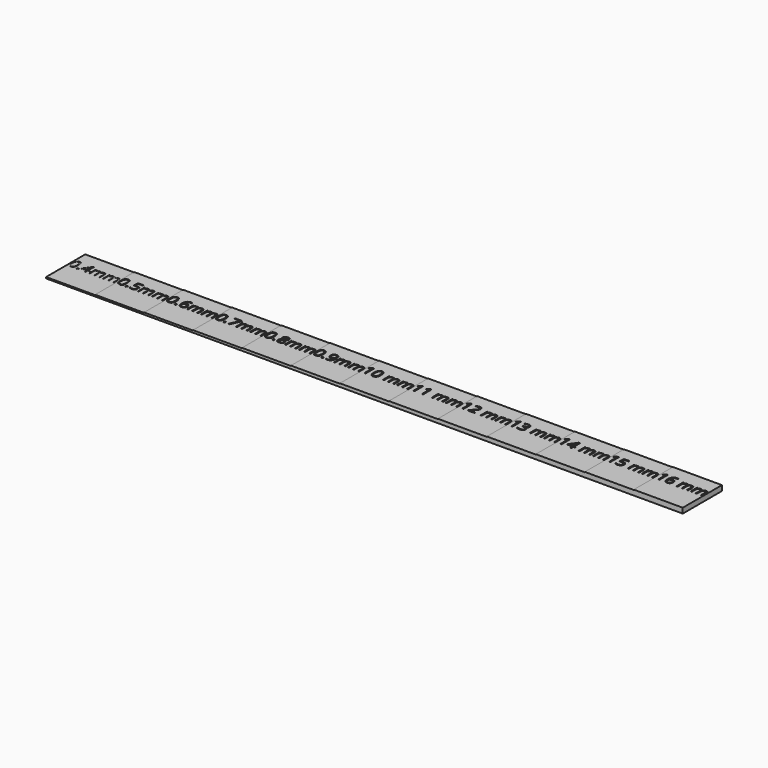
from build123d import *

# Parameters (mm, degrees)
F0_W          = 15
F0_H          = 15
F1_DEPTH      = 0.4
F2_DEPTH      = 0.5
F3_DEPTH      = 0.6
F4_DEPTH      = 0.7
F5_DEPTH      = 0.8
F6_DEPTH      = 0.9
F7_DEPTH      = 1
F8_DEPTH      = 1.1
F9_DEPTH      = 1.2
F10_DEPTH     = 1.3
F11_DEPTH     = 1.4
F12_DEPTH     = 1.5
F13_DEPTH     = 1.6
F14_TEXT_SIZE = 4.6102867022
F15_DEPTH     = 0.1
F16_TEXT_SIZE = 4.6102867022
F17_DEPTH     = 0.2
F18_TEXT_SIZE = 4.6102867022
F19_DEPTH     = 0.3
F20_TEXT_SIZE = 4.6102867022
F21_DEPTH     = 0.4
F22_TEXT_SIZE = 4.6102867022
F23_DEPTH     = 0.5
F24_TEXT_SIZE = 4.6102867022
F25_DEPTH     = 0.6
F26_TEXT_SIZE = 4.6191598903
F27_DEPTH     = 0.7
F28_TEXT_SIZE = 4.6191598903
F29_DEPTH     = 0.8
F30_TEXT_SIZE = 4.6191598903
F31_DEPTH     = 0.9
F32_TEXT_SIZE = 4.6191598903
F33_DEPTH     = 1
F34_TEXT_SIZE = 4.6191598903
F35_DEPTH     = 1.1
F36_TEXT_SIZE = 4.6191598903
F37_DEPTH     = 1.2
F38_TEXT_SIZE = 4.6191598903
F39_DEPTH     = 1.3


# Not quite as in the source:
# - Text() gives the source's letters only with a copy of the font that has no kerning and outlines rounded to 1/6400 em; it was checked with that copy


with BuildPart() as f1:
    # F0 (on Top) → F1 (new body)
    with BuildSketch(Plane.XY):
        with Locations((-77.3718157444, -0.2832734026)):
            Rectangle(F0_W, F0_H)
    extrude(amount=F1_DEPTH)

    # F0 (on Top) → F2 (join)
    with BuildSketch(Plane.XY):
        with Locations((-62.3718157444, -0.2832734026)):
            Rectangle(F0_W, F0_H)
    extrude(amount=F2_DEPTH)

    # F0 (on Top) → F3 (join)
    with BuildSketch(Plane.XY):
        with Locations((-47.3718157444, -0.2832734026)):
            Rectangle(F0_W, F0_H)
    extrude(amount=F3_DEPTH)

    # F0 (on Top) → F4 (join)
    with BuildSketch(Plane.XY):
        with Locations((-32.3718157444, -0.2832734026)):
            Rectangle(F0_W, F0_H)
    extrude(amount=F4_DEPTH)

    # F0 (on Top) → F5 (join)
    with BuildSketch(Plane.XY):
        with Locations((-17.3718157444, -0.2832734026)):
            Rectangle(F0_W, F0_H)
    extrude(amount=F5_DEPTH)

    # F0 (on Top) → F6 (join)
    with BuildSketch(Plane.XY):
        with Locations((-2.3718157444, -0.2832734026)):
            Rectangle(F0_W, F0_H)
    extrude(amount=F6_DEPTH)

    # F0 (on Top) → F7 (join)
    with BuildSketch(Plane.XY):
        with Locations((12.6281842556, -0.2832734026)):
            Rectangle(F0_W, F0_H)
    extrude(amount=F7_DEPTH)

    # F0 (on Top) → F8 (join)
    with BuildSketch(Plane.XY):
        with Locations((27.6281842556, -0.2832734026)):
            Rectangle(F0_W, F0_H)
    extrude(amount=F8_DEPTH)

    # F0 (on Top) → F9 (join)
    with BuildSketch(Plane.XY):
        with Locations((42.6281842556, -0.2832734026)):
            Rectangle(F0_W, F0_H)
    extrude(amount=F9_DEPTH)

    # F0 (on Top) → F10 (join)
    with BuildSketch(Plane.XY):
        with Locations((57.6281842556, -0.2832734026)):
            Rectangle(F0_W, F0_H)
    extrude(amount=F10_DEPTH)

    # F0 (on Top) → F11 (join)
    with BuildSketch(Plane.XY):
        with Locations((72.6281842556, -0.2832734026)):
            Rectangle(F0_W, F0_H)
    extrude(amount=F11_DEPTH)

    # F0 (on Top) → F12 (join)
    with BuildSketch(Plane.XY):
        with Locations((87.6281842556, -0.2832734026)):
            Rectangle(F0_W, F0_H)
    extrude(amount=F12_DEPTH)

    # F0 (on Top) → F13 (join)
    with BuildSketch(Plane.XY):
        with Locations((102.6281842556, -0.2832734026)):
            Rectangle(F0_W, F0_H)
    extrude(amount=F13_DEPTH)

    # F14 (on face) → F15 (cut)
    with BuildSketch(Plane.XY.offset(0.4)):
        with Locations((-84.8718157444, 0)):
            Text('0.4mm', F14_TEXT_SIZE, font='Open Sans', text_align=(TextAlign.LEFT, TextAlign.BOTTOM))
    extrude(amount=-F15_DEPTH, mode=Mode.SUBTRACT)

    # F16 (on face) → F17 (cut)
    with BuildSketch(Plane.XY.offset(0.5)):
        with Locations((-69.8718157444, 0)):
            Text('0.5mm', F16_TEXT_SIZE, font='Open Sans', text_align=(TextAlign.LEFT, TextAlign.BOTTOM))
    extrude(amount=-F17_DEPTH, mode=Mode.SUBTRACT)

    # F18 (on face) → F19 (cut)
    with BuildSketch(Plane.XY.offset(0.6)):
        with Locations((-54.8718157444, 0)):
            Text('0.6mm', F18_TEXT_SIZE, font='Open Sans', text_align=(TextAlign.LEFT, TextAlign.BOTTOM))
    extrude(amount=-F19_DEPTH, mode=Mode.SUBTRACT)

    # F20 (on face) → F21 (cut)
    with BuildSketch(Plane.XY.offset(0.7)):
        with Locations((-39.8718157444, 0)):
            Text('0.7mm', F20_TEXT_SIZE, font='Open Sans', text_align=(TextAlign.LEFT, TextAlign.BOTTOM))
    extrude(amount=-F21_DEPTH, mode=Mode.SUBTRACT)

    # F22 (on face) → F23 (cut)
    with BuildSketch(Plane.XY.offset(0.8)):
        with Locations((-24.8718157444, 0)):
            Text('0.8mm', F22_TEXT_SIZE, font='Open Sans', text_align=(TextAlign.LEFT, TextAlign.BOTTOM))
    extrude(amount=-F23_DEPTH, mode=Mode.SUBTRACT)

    # F24 (on face) → F25 (cut)
    with BuildSketch(Plane.XY.offset(0.9)):
        with Locations((-9.8718157444, 0)):
            Text('0.9mm', F24_TEXT_SIZE, font='Open Sans', text_align=(TextAlign.LEFT, TextAlign.BOTTOM))
    extrude(amount=-F25_DEPTH, mode=Mode.SUBTRACT)

    # F26 (on face) → F27 (cut)
    with BuildSketch(Plane.XY.offset(1)):
        with Locations((5.1281842556, 0)):
            Text('10 mm', F26_TEXT_SIZE, font='Open Sans', text_align=(TextAlign.LEFT, TextAlign.BOTTOM))
    extrude(amount=-F27_DEPTH, mode=Mode.SUBTRACT)

    # F28 (on face) → F29 (cut)
    with BuildSketch(Plane.XY.offset(1.1)):
        with Locations((20.1281842556, 0)):
            Text('11 mm', F28_TEXT_SIZE, font='Open Sans', text_align=(TextAlign.LEFT, TextAlign.BOTTOM))
    extrude(amount=-F29_DEPTH, mode=Mode.SUBTRACT)

    # F30 (on face) → F31 (cut)
    with BuildSketch(Plane.XY.offset(1.2)):
        with Locations((35.1281842556, 0)):
            Text('12 mm', F30_TEXT_SIZE, font='Open Sans', text_align=(TextAlign.LEFT, TextAlign.BOTTOM))
    extrude(amount=-F31_DEPTH, mode=Mode.SUBTRACT)

    # F32 (on face) → F33 (cut)
    with BuildSketch(Plane.XY.offset(1.3)):
        with Locations((50.1281842556, 0)):
            Text('13 mm', F32_TEXT_SIZE, font='Open Sans', text_align=(TextAlign.LEFT, TextAlign.BOTTOM))
    extrude(amount=-F33_DEPTH, mode=Mode.SUBTRACT)

    # F34 (on face) → F35 (cut)
    with BuildSketch(Plane.XY.offset(1.4)):
        with Locations((65.1281842556, 0)):
            Text('14 mm', F34_TEXT_SIZE, font='Open Sans', text_align=(TextAlign.LEFT, TextAlign.BOTTOM))
    extrude(amount=-F35_DEPTH, mode=Mode.SUBTRACT)

    # F36 (on face) → F37 (cut)
    with BuildSketch(Plane.XY.offset(1.5)):
        with Locations((80.1281842556, 0)):
            Text('15 mm', F36_TEXT_SIZE, font='Open Sans', text_align=(TextAlign.LEFT, TextAlign.BOTTOM))
    extrude(amount=-F37_DEPTH, mode=Mode.SUBTRACT)

    # F38 (on face) → F39 (cut)
    with BuildSketch(Plane.XY.offset(1.6)):
        with Locations((95.1281842556, 0)):
            Text('16 mm', F38_TEXT_SIZE, font='Open Sans', text_align=(TextAlign.LEFT, TextAlign.BOTTOM))
    extrude(amount=-F39_DEPTH, mode=Mode.SUBTRACT)


solid = f1.part
